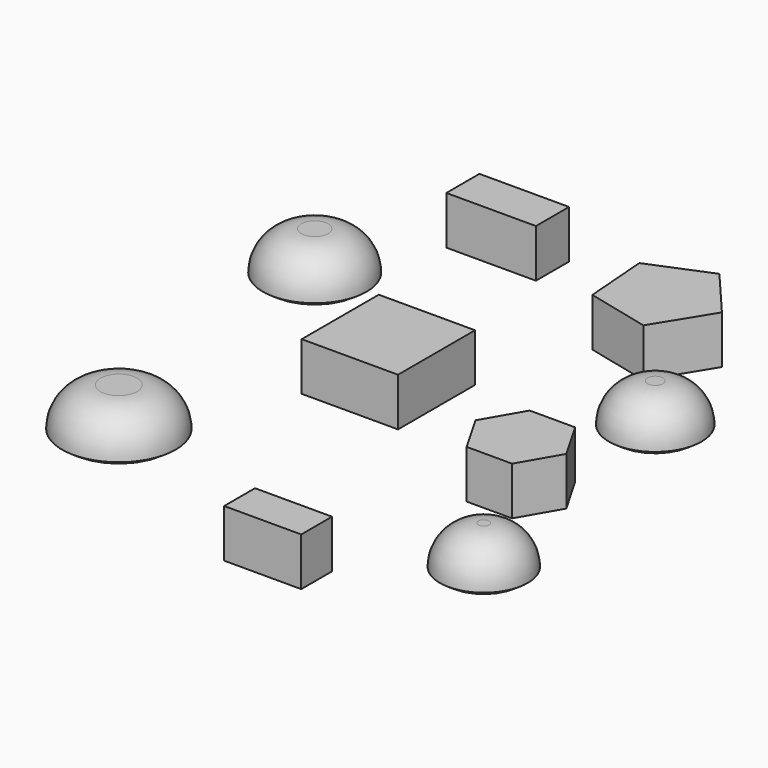
from build123d import *

# Parameters (mm, degrees)
F2_R      = 6.8511360946
F4_DEPTH  = 6.35
F1_R      = 6.1074642517
F3_R      = 7.4939547569
F0_R      = 5.7933229862
F5_R      = 5.08
F5_2_R    = 5.08
F5_3_R    = 5.08
F5_4_R    = 5.08
F11_W     = 11.8150338531
F11_H     = 5.45655936
F12_DEPTH = 6.35
F7_W      = 12.7
F7_H      = 12.7
F8_W      = 10.16
F8_H      = 5.08


# Not quite as in the source:
# - a fillet or chamfer that OpenCascade refuses, or shapes differently, is made with other operations: its cross-section is extruded or revolved along the edge and cut away or added


with BuildPart() as f4:
    # F2 (on Top) → F4 (new body)
    with BuildSketch(Plane.XY):
        with Locations((-29.0807504207, 15.4936052859)):
            Circle(F2_R)
    extrude(amount=F4_DEPTH)

    # F5
    f5_edges = [f4.edges().sort_by_distance(p)[0] for p in [
        (-35.931887, 15.493605, 6.35),
    ]]
    fillet(f5_edges, radius=F5_R)

    # F6: fillet of radius 5.08 on 1 edges, made by hand

    # F6_s1 → F6_t2 (revolve, cut)
    with BuildSketch(Plane.XZ.offset(-15.4936052859)):
        with BuildLine():
            ThreePointArc((-22.229614326, 1.27), (-23.7936672669, 0.3280951188), (-25.5897184911, 0))
            Line((-25.5897184911, 0), (-25.5897184911, -0.1016))
            Line((-25.5897184911, -0.1016), (-22.229614326, -0.1016))
            Line((-22.229614326, -0.1016), (-22.128014326, 0))
            ThreePointArc((-22.128014326, 0), (-22.128014326, 0.635), (-22.1624122427, 1.1938))
            Line((-22.1624122427, 1.1938), (-22.229614326, 1.27))
        make_face()
    revolve(axis=Axis((-29.0807504207, 15.4936052859, 0), (0, 0, 1)), mode=Mode.SUBTRACT)


with BuildPart() as f4b:
    # F1 (on Top) → F4, piece 2 (new body)
    with BuildSketch(Plane.XY):
        with Locations((19.489178434, 10.919265449)):
            Circle(F1_R)
    extrude(amount=F4_DEPTH)

    # F5#2
    f5_2_edges = [f4b.edges().sort_by_distance(p)[0] for p in [
        (13.381714, 10.919265, 6.35),
    ]]
    fillet(f5_2_edges, radius=F5_2_R)

    # F6#2: fillet of radius 5.08 on 1 edges, made by hand

    # F6_2_s1 → F6_2_t2 (revolve, cut)
    with BuildSketch(Plane.XZ.offset(-10.919265449)):
        with BuildLine():
            ThreePointArc((25.5966426857, 1.27), (24.0325897449, 0.3280951188), (22.2365385206, 0))
            Line((22.2365385206, 0), (22.2365385206, -0.1016))
            Line((22.2365385206, -0.1016), (25.5966426857, -0.1016))
            Line((25.5966426857, -0.1016), (25.6982426857, 0))
            ThreePointArc((25.6982426857, 0), (25.6982426857, 0.635), (25.663844769, 1.1938))
            Line((25.663844769, 1.1938), (25.5966426857, 1.27))
        make_face()
    revolve(axis=Axis((19.489178434, 10.919265449, 0), (0, 0, 1)), mode=Mode.SUBTRACT)


with BuildPart() as f4c:
    # F3 (on Top) → F4, piece 3 (new body)
    with BuildSketch(Plane.XY):
        with Locations((-23.076152429, -24.3060328066)):
            Circle(F3_R)
    extrude(amount=F4_DEPTH)

    # F5#3
    f5_3_edges = [f4c.edges().sort_by_distance(p)[0] for p in [
        (-30.570107, -24.306033, 6.35),
    ]]
    fillet(f5_3_edges, radius=F5_3_R)

    # F6#3: fillet of radius 5.08 on 1 edges, made by hand

    # F6_3_s1 → F6_3_t2 (revolve, cut)
    with BuildSketch(Plane.XZ.offset(24.3060328066)):
        with BuildLine():
            ThreePointArc((-15.5821976721, 1.27), (-17.1462506129, 0.3280951188), (-18.9423018371, 0))
            Line((-18.9423018371, 0), (-18.9423018371, -0.1016))
            Line((-18.9423018371, -0.1016), (-15.5821976721, -0.1016))
            Line((-15.5821976721, -0.1016), (-15.4805976721, 0))
            ThreePointArc((-15.4805976721, 0), (-15.4805976721, 0.635), (-15.5149955888, 1.1938))
            Line((-15.5149955888, 1.1938), (-15.5821976721, 1.27))
        make_face()
    revolve(axis=Axis((-23.076152429, -24.3060328066, 0), (0, 0, 1)), mode=Mode.SUBTRACT)


with BuildPart() as f4d:
    # F0 (on Top) → F4, piece 4 (new body)
    with BuildSketch(Plane.XY):
        with Locations((25.5116987973, -24.8762052506)):
            Circle(F0_R)
    extrude(amount=F4_DEPTH)

    # F5#4
    f5_4_edges = [f4d.edges().sort_by_distance(p)[0] for p in [
        (19.718376, -24.876205, 6.35),
    ]]
    fillet(f5_4_edges, radius=F5_4_R)

    # F6#4: fillet of radius 5.08 on 1 edges, made by hand

    # F6_4_s1 → F6_4_t2 (revolve, cut)
    with BuildSketch(Plane.XZ.offset(24.8762052506)):
        with BuildLine():
            ThreePointArc((31.3050217835, 1.27), (29.7409688427, 0.3280951188), (27.9449176185, 0))
            Line((27.9449176185, 0), (27.9449176185, -0.1016))
            Line((27.9449176185, -0.1016), (31.3050217835, -0.1016))
            Line((31.3050217835, -0.1016), (31.4066217835, 0))
            ThreePointArc((31.4066217835, 0), (31.4066217835, 0.635), (31.3722238668, 1.1938))
            Line((31.3722238668, 1.1938), (31.3050217835, 1.27))
        make_face()
    revolve(axis=Axis((25.5116987973, -24.8762052506, 0), (0, 0, 1)), mode=Mode.SUBTRACT)


with BuildPart() as f12:
    # F11 (on Top) → F12 (new body)
    with BuildSketch(Plane.XY):
        with Locations((-17.5771228969, 32.9260975122)):
            Rectangle(F11_W, F11_H)
    extrude(amount=F12_DEPTH)


with BuildPart() as f12b:
    # F10 (on Top) → F12, piece 2 (new body)
    with BuildSketch(Plane.XY):
        Polygon((15.3152750432, 27.1318872107), (9.7473977506, 33.6748863922), (1.8040670369, 30.4014183524), (2.4626959646, 21.8353046612), (10.8130817416, 19.8146232884), align=None)
    extrude(amount=F12_DEPTH)


with BuildPart() as f12c:
    # F7 (on Top) → F12, piece 3 (new body)
    with BuildSketch(Plane.XY):
        with Locations((-8.3940104418, 1.7794129275)):
            Rectangle(F7_W, F7_H)
    extrude(amount=F12_DEPTH)


with BuildPart() as f12d:
    # F9 (on Top) → F12, piece 4 (new body)
    with BuildSketch(Plane.XY):
        Polygon((13.5294110343, -12.7222305164), (19.5252872243, -12.7222305164), (22.5232253194, -7.5296494178), (19.5252872243, -2.3370683193), (13.5294110343, -2.3370683193), (10.5314729393, -7.5296494178), align=None)
    extrude(amount=F12_DEPTH)


with BuildPart() as f12e:
    # F8 (on Top) → F12, piece 5 (new body)
    with BuildSketch(Plane.XY):
        with Locations((7.3472648245, -36.0771489954)):
            Rectangle(F8_W, F8_H)
    extrude(amount=F12_DEPTH)


solid = Compound([f4.part, f4b.part, f4c.part, f4d.part, f12.part, f12b.part, f12c.part, f12d.part, f12e.part])
